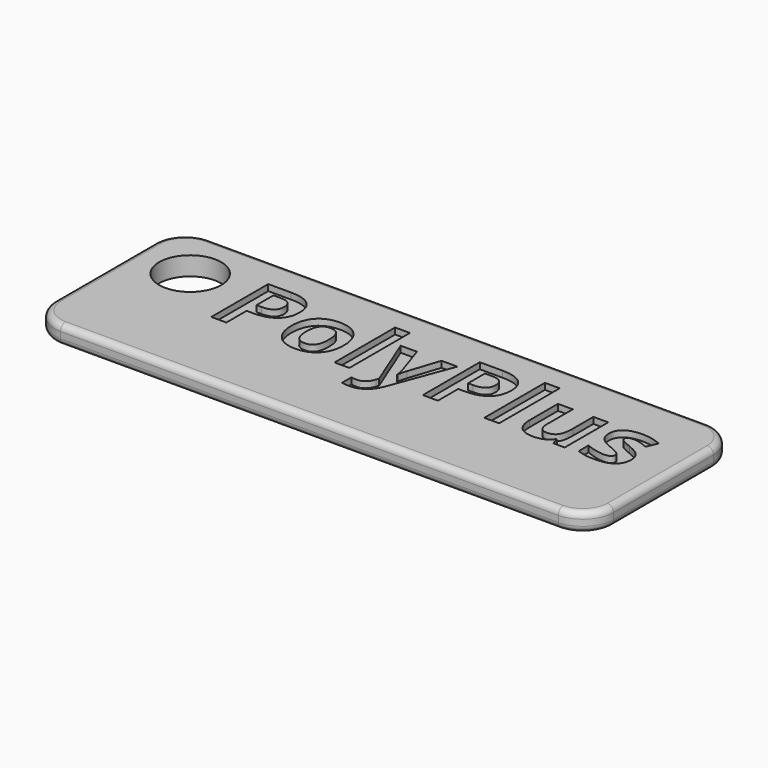
from build123d import *

# Parameters (mm, degrees)
F0_W         = 90
F0_H         = 30
F1_DEPTH     = 3
F2_R         = 1
F3_T1_DEPTH  = 3
F3_T4_ANGLE  = 90
F3_T6_ANGLE  = 90
F3_T8_ANGLE  = 90
F3_T10_ANGLE = 90
F3_T12_ANGLE = 90
F3_T14_ANGLE = 90
F3_T16_ANGLE = 90
F3_T18_ANGLE = 90
F4_R         = 5
F5_DEPTH     = 3
F6_TEXT_SIZE = 16.0548935699
F7_DEPTH     = 1


# Not quite as in the source:
# - a fillet or chamfer that OpenCascade refuses, or shapes differently, is made with other operations: its cross-section is extruded or revolved along the edge and cut away or added
# - Text() gives the source's letters only with a copy of the font that has no kerning and outlines rounded to 1/6400 em; it was checked with that copy


with BuildPart() as f1:
    # F0 (on Top) → F1 (new body)
    with BuildSketch(Plane.XY):
        Rectangle(F0_W, F0_H)
    extrude(amount=F1_DEPTH)

    # F2
    f2_edges = [f1.edges().sort_by_distance(p)[0] for p in [
        (0, 15, 3),
        (-45, 0, 3),
        (0, -15, 3),
        (45, 0, 3),
        (0, 15, 0),
        (-45, 0, 0),
        (0, -15, 0),
        (45, 0, 0),
    ]]
    fillet(f2_edges, radius=F2_R)

    # F3: fillet of radius 5 on 4 edges, made by hand

    # F3_s2 → F3_t1 (cut)
    with BuildSketch(Plane.XY):
        with BuildLine():
            ThreePointArc((45.0004, -9.9990343146), (43.5355339059, -13.5355339059), (39.9990343146, -15.0004))
            Line((39.9990343146, -15.0004), (39.9990343146, -15.5005365685))
            ThreePointArc((39.9990343146, -15.5005365685), (42.4995171573, -15.5001365685), (45, -15.5001365685))
            Line((45, -15.5001365685), (45.5001365685, -15))
            ThreePointArc((45.5001365685, -15), (45.5001365685, -12.4995171573), (45.5005365685, -9.9990343146))
            Line((45.5005365685, -9.9990343146), (45.0004, -9.9990343146))
        make_face()
        with BuildLine():
            ThreePointArc((39.9990343146, 15.0004), (43.5355339059, 13.5355339059), (45.0004, 9.9990343146))
            Line((45.0004, 9.9990343146), (45.5005365685, 9.9990343146))
            ThreePointArc((45.5005365685, 9.9990343146), (45.5001365685, 12.4995171573), (45.5001365685, 15))
            Line((45.5001365685, 15), (45, 15.5001365685))
            ThreePointArc((45, 15.5001365685), (42.4995171573, 15.5001365685), (39.9990343146, 15.5005365685))
            Line((39.9990343146, 15.5005365685), (39.9990343146, 15.0004))
        make_face()
        with BuildLine():
            ThreePointArc((-39.9990343146, 15.0004), (-43.5355339059, 13.5355339059), (-45.0004, 9.9990343146))
            Line((-45.0004, 9.9990343146), (-45.5005365685, 9.9990343146))
            ThreePointArc((-45.5005365685, 9.9990343146), (-45.5001365685, 12.4995171573), (-45.5001365685, 15))
            Line((-45.5001365685, 15), (-45, 15.5001365685))
            ThreePointArc((-45, 15.5001365685), (-42.4995171573, 15.5001365685), (-39.9990343146, 15.5005365685))
            Line((-39.9990343146, 15.5005365685), (-39.9990343146, 15.0004))
        make_face()
        with BuildLine():
            ThreePointArc((-45.0004, -9.9990343146), (-43.5355339059, -13.5355339059), (-39.9990343146, -15.0004))
            Line((-39.9990343146, -15.0004), (-39.9990343146, -15.5005365685))
            ThreePointArc((-39.9990343146, -15.5005365685), (-42.4995171573, -15.5001365685), (-45, -15.5001365685))
            Line((-45, -15.5001365685), (-45.5001365685, -15))
            ThreePointArc((-45.5001365685, -15), (-45.5001365685, -12.4995171573), (-45.5005365685, -9.9990343146))
            Line((-45.5005365685, -9.9990343146), (-45.0004, -9.9990343146))
        make_face()
    extrude(amount=F3_T1_DEPTH, mode=Mode.SUBTRACT)

    # F3_s3 → F3_t4 (revolve, cut)
    with BuildSketch(Plane.YZ.offset(-39.9990343146)):
        with BuildLine():
            ThreePointArc((-14.0004, 0), (-14.7075067812, 0.2928932188), (-15.0004, 1))
            Line((-15.0004, 1), (-15.0004, 0))
            Line((-15.0004, 0), (-14.0004, 0))
        make_face()
    revolve(axis=Axis((-39.9990343146, -9.9990343146, 0), (0, 0, -1)), revolution_arc=F3_T4_ANGLE, mode=Mode.SUBTRACT)

    # F3_s5 → F3_t6 (revolve, cut)
    with BuildSketch(Plane.XZ.offset(9.9990343146)):
        with BuildLine():
            ThreePointArc((-44.0004, 3), (-44.7075067812, 2.7071067812), (-45.0004, 2))
            Line((-45.0004, 2), (-45.0004, 3))
            Line((-45.0004, 3), (-44.0004, 3))
        make_face()
    revolve(axis=Axis((-39.9990343146, -9.9990343146, 3), (0, 0, 1)), revolution_arc=F3_T6_ANGLE, mode=Mode.SUBTRACT)

    # F3_s7 → F3_t8 (revolve, cut)
    with BuildSketch(Plane.XZ.offset(-9.9990343146)):
        with BuildLine():
            ThreePointArc((-44.0004, 0), (-44.7075067812, 0.2928932188), (-45.0004, 1))
            Line((-45.0004, 1), (-45.0004, 0))
            Line((-45.0004, 0), (-44.0004, 0))
        make_face()
    revolve(axis=Axis((-39.9990343146, 9.9990343146, 0), (0, 0, -1)), revolution_arc=F3_T8_ANGLE, mode=Mode.SUBTRACT)

    # F3_s9 → F3_t10 (revolve, cut)
    with BuildSketch(Plane.YZ.offset(-39.9990343146)):
        with BuildLine():
            ThreePointArc((14.0004, 3), (14.7075067812, 2.7071067812), (15.0004, 2))
            Line((15.0004, 2), (15.0004, 3))
            Line((15.0004, 3), (14.0004, 3))
        make_face()
    revolve(axis=Axis((-39.9990343146, 9.9990343146, 3), (0, 0, 1)), revolution_arc=F3_T10_ANGLE, mode=Mode.SUBTRACT)

    # F3_s11 → F3_t12 (revolve, cut)
    with BuildSketch(Plane.YZ.offset(39.9990343146)):
        with BuildLine():
            ThreePointArc((14.0004, 0), (14.7075067812, 0.2928932188), (15.0004, 1))
            Line((15.0004, 1), (15.0004, 0))
            Line((15.0004, 0), (14.0004, 0))
        make_face()
    revolve(axis=Axis((39.9990343146, 9.9990343146, 0), (0, 0, -1)), revolution_arc=F3_T12_ANGLE, mode=Mode.SUBTRACT)

    # F3_s13 → F3_t14 (revolve, cut)
    with BuildSketch(Plane.XZ.offset(-9.9990343146)):
        with BuildLine():
            ThreePointArc((44.0004, 3), (44.7075067812, 2.7071067812), (45.0004, 2))
            Line((45.0004, 2), (45.0004, 3))
            Line((45.0004, 3), (44.0004, 3))
        make_face()
    revolve(axis=Axis((39.9990343146, 9.9990343146, 3), (0, 0, 1)), revolution_arc=F3_T14_ANGLE, mode=Mode.SUBTRACT)

    # F3_s15 → F3_t16 (revolve, cut)
    with BuildSketch(Plane.XZ.offset(9.9990343146)):
        with BuildLine():
            ThreePointArc((44.0004, 0), (44.7075067812, 0.2928932188), (45.0004, 1))
            Line((45.0004, 1), (45.0004, 0))
            Line((45.0004, 0), (44.0004, 0))
        make_face()
    revolve(axis=Axis((39.9990343146, -9.9990343146, 0), (0, 0, -1)), revolution_arc=F3_T16_ANGLE, mode=Mode.SUBTRACT)

    # F3_s17 → F3_t18 (revolve, cut)
    with BuildSketch(Plane.YZ.offset(39.9990343146)):
        with BuildLine():
            ThreePointArc((-14.0004, 3), (-14.7075067812, 2.7071067812), (-15.0004, 2))
            Line((-15.0004, 2), (-15.0004, 3))
            Line((-15.0004, 3), (-14.0004, 3))
        make_face()
    revolve(axis=Axis((39.9990343146, -9.9990343146, 3), (0, 0, 1)), revolution_arc=F3_T18_ANGLE, mode=Mode.SUBTRACT)

    # F4 (on face) → F5 (cut)
    with BuildSketch(Plane.XY.offset(3)):
        with Locations((-36, 6)):
            Circle(F4_R)
    extrude(amount=-F5_DEPTH, mode=Mode.SUBTRACT)

    # F6 (on face) → F7 (cut)
    with BuildSketch(Plane.XY.offset(3)):
        with Locations((-28, -1.5595233703)):
            Text('PolyPlus', F6_TEXT_SIZE, font='Open Sans', font_style=FontStyle.BOLD, text_align=(TextAlign.LEFT, TextAlign.BOTTOM))
    extrude(amount=-F7_DEPTH, mode=Mode.SUBTRACT)


solid = f1.part
